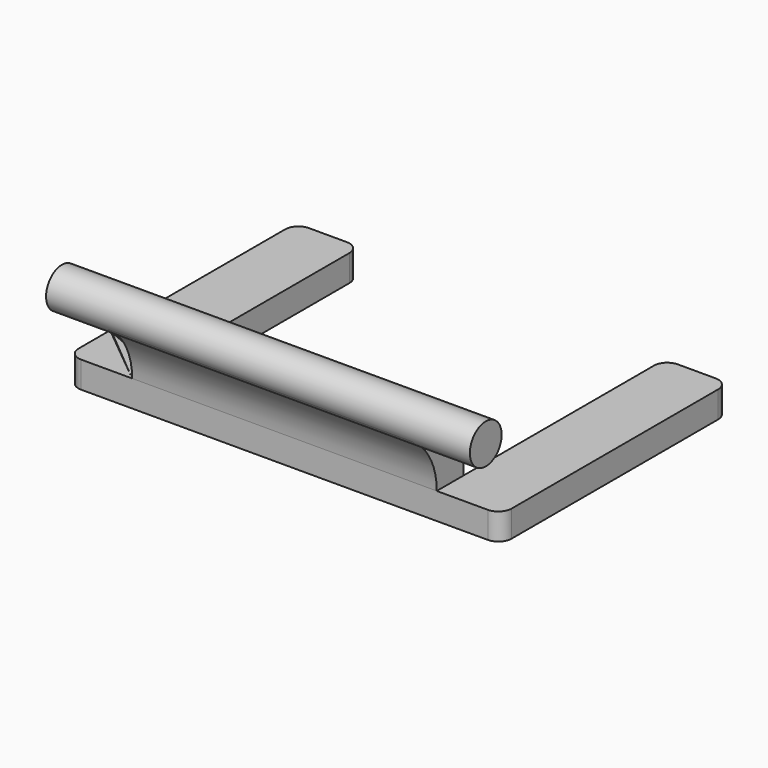
from build123d import *

# Parameters (mm, degrees)
F1_DEPTH     = 2
F2_W         = 23
F2_H         = 2.5
F3_DEPTH     = 5
F6_R         = 1.5
F7_DEPTH     = 32
F9_DEPTH     = 23
F10_T1_DEPTH = 43


# Not quite as in the source:
# - a fillet or chamfer that OpenCascade refuses, or shapes differently, is made with other operations: its cross-section is extruded or revolved along the edge and cut away or added


with BuildPart() as f1:
    # F0 (on Top) → F1 (new body)
    with BuildSketch(Plane.XY):
        with BuildLine():
            Line((-15.35, -10.75), (15.35, -10.75))
            ThreePointArc((15.35, -10.75), (16.057107, -10.457107), (16.35, -9.75))
            Line((16.35, -9.75), (16.35, 9.75))
            ThreePointArc((16.35, 9.75), (16.057107, 10.457107), (15.35, 10.75))
            Line((15.35, 10.75), (12.5, 10.75))
            ThreePointArc((12.5, 10.75), (11.792893, 10.457107), (11.5, 9.75))
            Line((11.5, 9.75), (11.5, -8.25))
            Line((11.5, -8.25), (-11.5, -8.25))
            Line((-11.5, -8.25), (-11.5, 9.75))
            ThreePointArc((-11.5, 9.75), (-11.792893, 10.457107), (-12.5, 10.75))
            Line((-12.5, 10.75), (-15.35, 10.75))
            ThreePointArc((-15.35, 10.75), (-16.057107, 10.457107), (-16.35, 9.75))
            Line((-16.35, 9.75), (-16.35, -9.75))
            ThreePointArc((-16.35, -9.75), (-16.057107, -10.457107), (-15.35, -10.75))
        make_face()
    extrude(amount=F1_DEPTH)

    # F2 (on face) → F3 (join)
    with BuildSketch(Plane.XY.offset(2)):
        with Locations((0, -9.5)):
            Rectangle(F2_W, F2_H)
    extrude(amount=F3_DEPTH)

    # F6 (on offset) → F7 (join, through all)
    with BuildSketch(Plane.YZ.offset(16)):
        with Locations((-11.75, 7)):
            Circle(F6_R)
    extrude(amount=-F7_DEPTH)

    # F8 (on face) → F9 (join, through all)
    with BuildSketch(Plane.YZ.offset(11.5)):
        with BuildLine():
            ThreePointArc((-10.25, 7), (-12.177978, 8.437649), (-13.00578, 6.179624))
            Line((-13.00578, 6.179624), (-10.75, 6.179624))
            Line((-10.75, 6.179624), (-10.75, 5.881966))
            ThreePointArc((-10.75, 5.881966), (-10.380694, 6.387628), (-10.25, 7))
        make_face()
        with BuildLine():
            ThreePointArc((-12.274708, 5.594766), (-12.626525, 5.904344), (-13.00578, 6.179624))
            ThreePointArc((-13.00578, 6.179624), (-12.687043, 5.828697), (-12.274708, 5.594766))
        make_face()
        with BuildLine():
            Line((-10.75, 6.179624), (-13.00578, 6.179624))
            ThreePointArc((-13.00578, 6.179624), (-12.626525, 5.904344), (-12.274708, 5.594766))
            ThreePointArc((-12.274708, 5.594766), (-11.472337, 5.525923), (-10.75, 5.881966))
            Line((-10.75, 5.881966), (-10.75, 6.179624))
        make_face()
        with BuildLine():
            ThreePointArc((-10.75, 5.881966), (-11.472337, 5.525923), (-12.274708, 5.594766))
            ThreePointArc((-12.274708, 5.594766), (-11.146933, 3.952375), (-10.75, 2))
            Line((-10.75, 2), (-10.75, 5.881966))
        make_face()
    extrude(amount=-F9_DEPTH)

    # F10: fillet of radius 5 on 1 edges, made by hand

    # F10_s2 → F10_t1 (cut)
    with BuildSketch(Plane.YZ.offset(-21.5)):
        with BuildLine():
            ThreePointArc((-8.25, 3), (-8.777864, 5.236068), (-10.25, 7))
            Line((-10.25, 7), (-10.19, 7.08))
            ThreePointArc((-10.19, 7.08), (-9.25, 7.1), (-8.25, 7.1))
            Line((-8.25, 7.1), (-8.15, 7))
            Line((-8.15, 7), (-8.15, 3))
            Line((-8.15, 3), (-8.25, 3))
        make_face()
    extrude(amount=F10_T1_DEPTH, mode=Mode.SUBTRACT)


solid = f1.part
